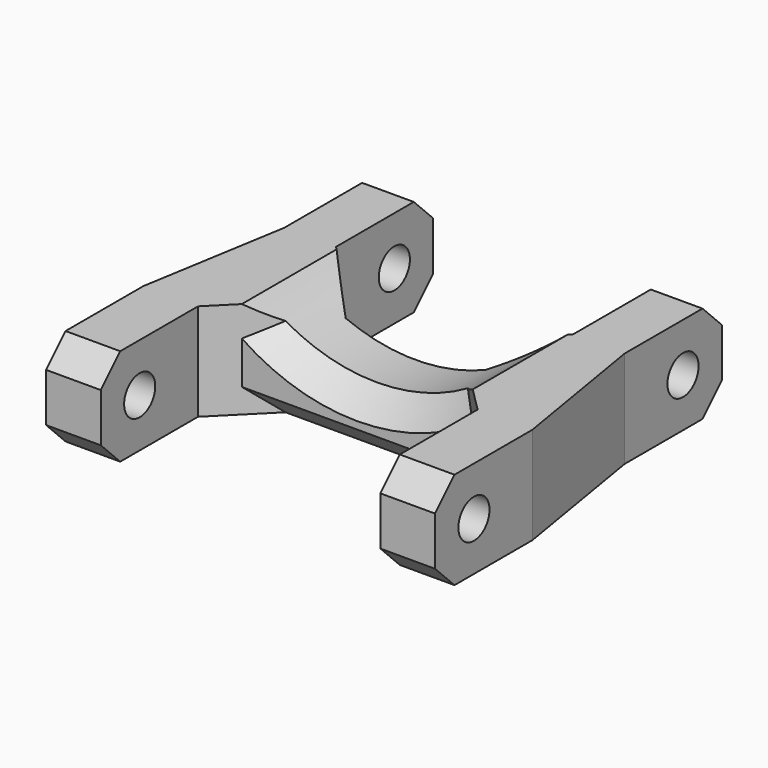
from build123d import *

# Parameters (mm, degrees)
F1_DEPTH      = 8
F2_W          = 19.5
F2_H          = 12
F2_W_2        = 23
F3_DEPTH      = 8
F4_R          = 1.6
F5_DEPTH      = 32
F6_R          = 1.6
F7_DEPTH      = 28
F8_SIZE       = 2
F10_DEPTH     = 9.751
F11_T1_DEPTH  = 14.7867319519
F11_T3_DEPTH  = 14.7867319519
F11_T5_DEPTH  = 14.5367319519
F11_T7_DEPTH  = 14.5367319519
F11_T12_DEPTH = 25.7867319519
F11_T18_DEPTH = 29.2867319519
F11_T24_ANGLE = 117.8974179381
F11_T30_ANGLE = 101.5178089871


# Not quite as in the source:
# - a fillet or chamfer that OpenCascade refuses, or shapes differently, is made with other operations: its cross-section is extruded or revolved along the edge and cut away or added


with BuildPart() as f1:
    # F0 (on Top) → F1 (new body)
    with BuildSketch(Plane.XY):
        Polygon((14, 22), (-14, 22), (-14, 12), (-16, 0), (-16, -10), (16, -10), (16, 0), (14, 12), align=None)
    extrude(amount=F1_DEPTH)

    # F2 (on face) → F3 (cut, through all)
    with BuildSketch(Plane.XY.offset(8)):
        with Locations((0, 16)):
            Rectangle(F2_W, F2_H)
        with Locations((0, -4)):
            Rectangle(F2_W_2, F2_H)
    extrude(amount=-F3_DEPTH, mode=Mode.SUBTRACT)

    # F4 (on face) → F5 (cut, through all)
    with BuildSketch(Plane.YZ.offset(16)):
        with Locations((-6, 4)):
            Circle(F4_R)
    extrude(amount=-F5_DEPTH, mode=Mode.SUBTRACT)

    # F6 (on face) → F7 (cut, through all)
    with BuildSketch(Plane.YZ.offset(14)):
        with Locations((18, 4)):
            Circle(F6_R)
    extrude(amount=-F7_DEPTH, mode=Mode.SUBTRACT)

    # F8
    f8_edges = [f1.edges().sort_by_distance(p)[0] for p in [
        (9.75, 10, 4),
        (-9.75, 10, 4),
        (11.5, 2, 4),
        (-11.5, 2, 4),
    ]]
    chamfer(f8_edges, length=F8_SIZE)

    # F9 (on face) → F10 (cut, through all)
    with BuildSketch(Plane.XZ.offset(-2)):
        with BuildLine():
            Line((9.5, 8), (-9.5, 8))
            ThreePointArc((-9.5, 8), (0, 4.6081867662), (9.5, 8))
        make_face()
    extrude(amount=-F10_DEPTH, mode=Mode.SUBTRACT)

    # F11: chamfer of 2 on 12 edges, made by hand

    # F11_s2 → F11_t1 (cut)
    with BuildSketch(Plane.YZ.offset(-21.1433659759)):
        Polygon((-10, 6), (-8, 8), (-10, 8), align=None)
        Polygon((-8, 0), (-10, 2), (-10, 0), align=None)
    extrude(amount=F11_T1_DEPTH, mode=Mode.SUBTRACT)

    # F11_s4 → F11_t3 (cut)
    with BuildSketch(Plane.YZ.offset(6.3566340241)):
        Polygon((-10, 6), (-8, 8), (-10, 8), align=None)
        Polygon((-8, 0), (-10, 2), (-10, 0), align=None)
    extrude(amount=F11_T3_DEPTH, mode=Mode.SUBTRACT)

    # F11_s6 → F11_t5 (cut)
    with BuildSketch(Plane.YZ.offset(4.6066340241)):
        Polygon((22, 6), (20, 8), (22, 8), align=None)
        Polygon((20, 0), (22, 2), (22, 0), align=None)
    extrude(amount=F11_T5_DEPTH, mode=Mode.SUBTRACT)

    # F11_s8 → F11_t7 (cut)
    with BuildSketch(Plane.YZ.offset(-19.1433659759)):
        Polygon((20, 0), (22, 2), (22, 0), align=None)
        Polygon((22, 6), (20, 8), (22, 8), align=None)
    extrude(amount=F11_T7_DEPTH, mode=Mode.SUBTRACT)


with BuildPart() as f11_tool10:
    # F11_s11 → F11_t12 (new body)
    with BuildSketch(Plane.YZ.offset(-12.8933659759)):
        Polygon((8, 0), (10, 2), (10, 0), align=None)
    extrude(amount=F11_T12_DEPTH)

    split(bisect_by=Plane(origin=(-1.125, 1.125, 0), x_dir=(0, 0, 1), z_dir=(-0.7071067812, 0.7071067812, 0)), keep=Keep.TOP)

    split(bisect_by=Plane(origin=(1.125, 1.125, 0), x_dir=(0, 0, 1), z_dir=(0.7071067812, 0.7071067812, 0)), keep=Keep.TOP)


with BuildPart() as f1_1:
    add(f1.part)

    # F11_t9: cut F11_tool10
    add(f11_tool10.part, mode=Mode.SUBTRACT)


with BuildPart() as f11_tool16:
    # F11_s17 → F11_t18 (new body)
    with BuildSketch(Plane.YZ.offset(14.6433659759)):
        Polygon((4, 0), (2, 2), (2, 0), align=None)
    extrude(amount=-F11_T18_DEPTH)

    split(bisect_by=Plane(origin=(5.75, 5.75, 0), x_dir=(0, 0, 1), z_dir=(-0.7071067812, -0.7071067812, 0)), keep=Keep.TOP)

    split(bisect_by=Plane(origin=(-5.75, 5.75, 0), x_dir=(0, 0, 1), z_dir=(0.7071067812, -0.7071067812, 0)), keep=Keep.TOP)


with BuildPart() as f1_2:
    add(f1_1.part)

    # F11_t15: cut F11_tool16
    add(f11_tool16.part, mode=Mode.SUBTRACT)


with BuildPart() as f11_tool22:
    # F11_s23 → F11_t24 (revolve)
    with BuildSketch(Plane(origin=(-8.664727501, 0, 14.3913305034), x_dir=(0, 1, 0), z_dir=(-0.5158052023, 0, 0.8567058966))):
        Polygon((2, 6.8859952574), (4, 4.8859952574), (2, 4.8859952574), align=None)
    revolve(axis=Axis((0, 2, 19.6081867662), (0, -1, 0)), revolution_arc=F11_T24_ANGLE)

    split(bisect_by=Plane(origin=(5.75, 5.75, 0), x_dir=(0, 0, 1), z_dir=(-0.7071067812, -0.7071067812, 0)), keep=Keep.TOP)

    split(bisect_by=Plane(origin=(-5.75, 5.75, 0), x_dir=(0, 0, 1), z_dir=(0.7071067812, -0.7071067812, 0)), keep=Keep.TOP)


with BuildPart() as f1_3:
    add(f1_2.part)

    # F11_t21: cut F11_tool22
    add(f11_tool22.part, mode=Mode.SUBTRACT)


with BuildPart() as f11_tool28:
    # F11_s29 → F11_t30 (revolve)
    with BuildSketch(Plane(origin=(-9.6066653022, 0, 11.7617013204), x_dir=(0, 1, 0), z_dir=(-0.6325849704, 0, 0.7744909652))):
        Polygon((10, 4.596155754), (8, 2.596155754), (10, 2.596155754), align=None)
    revolve(axis=Axis((0, 10, 19.6081867662), (0, -1, 0)), revolution_arc=F11_T30_ANGLE)

    split(bisect_by=Plane(origin=(-1.125, 1.125, 0), x_dir=(0, 0, 1), z_dir=(-0.7071067812, 0.7071067812, 0)), keep=Keep.TOP)

    split(bisect_by=Plane(origin=(1.125, 1.125, 0), x_dir=(0, 0, 1), z_dir=(0.7071067812, 0.7071067812, 0)), keep=Keep.TOP)


with BuildPart() as f1_4:
    add(f1_3.part)

    # F11_t27: cut F11_tool28
    add(f11_tool28.part, mode=Mode.SUBTRACT)


solid = f1_4.part
